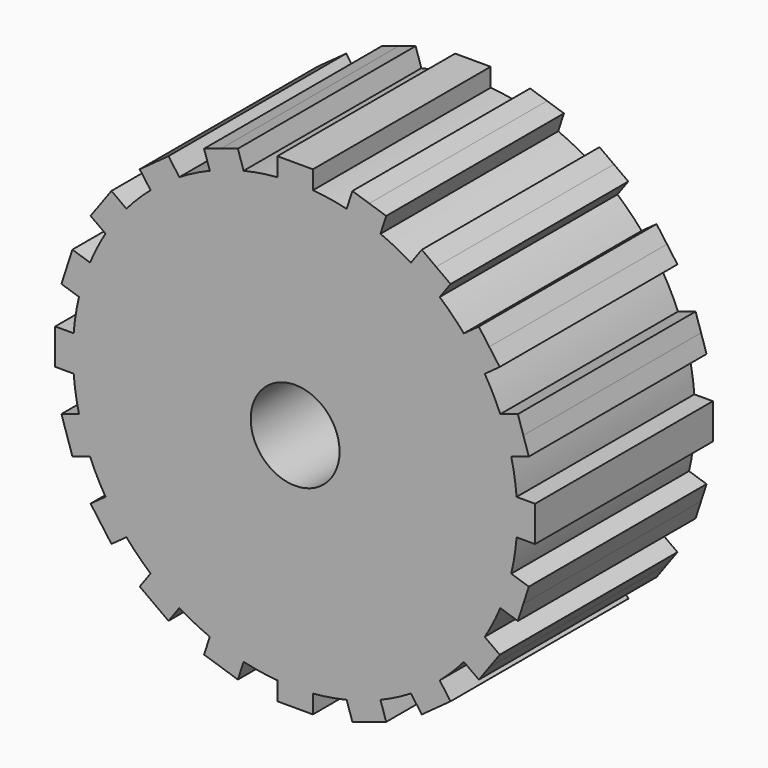
from build123d import *

# Parameters (mm, degrees)
F0_R     = 1.27
F1_DEPTH = 6.35


# Not quite as in the source:
# - a feature names something its author has since deleted; it is built from what else it names


with BuildPart() as f1:
    # F0 (on Front) → F1 (new body)
    with BuildSketch(Plane.XZ):
        with BuildLine():
            ThreePointArc((-2.4391053202, 5.8628717568), (-1.9622579143, 6.0392088785), (-1.4728318996, 6.1768330231))
            Line((-1.4728318996, 6.1768330231), (-1.6361018371, 6.6793262219))
            Line((-1.6361018371, 6.6793262219), (-2.1192385474, 6.5223455888))
            Line((-2.1192385474, 6.5223455888), (-2.6023752577, 6.3653649556))
            Line((-2.6023752577, 6.3653649556), (-2.4391053202, 5.8628717568))
        make_face()
        with BuildLine():
            ThreePointArc((-0.508, 6.3296473835), (-0.2542037711, 6.3449098057), (0, 6.35))
            Line((0, 6.35), (0, 6.858))
            Line((0, 6.858), (-0.508, 6.858))
            Line((-0.508, 6.858), (-0.508, 6.3296473835))
        make_face()
        with BuildLine():
            ThreePointArc((0, 6.35), (0.2542037711, 6.3449098057), (0.508, 6.3296473835))
            Line((0.508, 6.3296473835), (0.508, 6.858))
            Line((0.508, 6.858), (0, 6.858))
            Line((0, 6.858), (0, 6.35))
        make_face()
        with BuildLine():
            ThreePointArc((1.4728318996, 6.1768330231), (1.9622579143, 6.0392088785), (2.4391053202, 5.8628717568))
            Line((2.4391053202, 5.8628717568), (2.6023752577, 6.3653649556))
            Line((2.6023752577, 6.3653649556), (2.1192385474, 6.5223455888))
            Line((2.1192385474, 6.5223455888), (1.6361018371, 6.6793262219))
            Line((1.6361018371, 6.6793262219), (1.4728318996, 6.1768330231))
        make_face()
        with BuildLine():
            ThreePointArc((3.3094927511, 5.4193872099), (3.7324363521, 5.1372579143), (4.1314540174, 4.8221973935))
            Line((4.1314540174, 4.8221973935), (4.4420118934, 5.2496436393))
            Line((4.4420118934, 5.2496436393), (4.0310312602, 5.5482385474))
            Line((4.0310312602, 5.5482385474), (3.6200506271, 5.8468334556))
            Line((3.6200506271, 5.8468334556), (3.3094927511, 5.4193872099))
        make_face()
        with BuildLine():
            ThreePointArc((4.8221973935, 4.1314540174), (5.1372579143, 3.7324363521), (5.4193872099, 3.3094927511))
            Line((5.4193872099, 3.3094927511), (5.8468334556, 3.6200506271))
            Line((5.8468334556, 3.6200506271), (5.5482385474, 4.0310312602))
            Line((5.5482385474, 4.0310312602), (5.2496436393, 4.4420118934))
            Line((5.2496436393, 4.4420118934), (4.8221973935, 4.1314540174))
        make_face()
        with BuildLine():
            Line((0.508, -6.858), (0.508, -6.3296473835))
            ThreePointArc((0.508, -6.3296473835), (0, -6.35), (-0.508, -6.3296473835))
            Line((-0.508, -6.3296473835), (-0.508, -6.858))
            Line((-0.508, -6.858), (0, -6.858))
            Line((0, -6.858), (0.508, -6.858))
        make_face()
        with BuildLine():
            Line((2.6023752577, -6.3653649556), (2.4391053202, -5.8628717568))
            ThreePointArc((2.4391053202, -5.8628717568), (1.9622579143, -6.0392088785), (1.4728318996, -6.1768330231))
            Line((1.4728318996, -6.1768330231), (1.6361018371, -6.6793262219))
            Line((1.6361018371, -6.6793262219), (2.1192385474, -6.5223455888))
            Line((2.1192385474, -6.5223455888), (2.6023752577, -6.3653649556))
        make_face()
        with BuildLine():
            Line((4.4420118934, -5.2496436393), (4.1314540174, -4.8221973935))
            ThreePointArc((4.1314540174, -4.8221973935), (3.7324363521, -5.1372579143), (3.3094927511, -5.4193872099))
            Line((3.3094927511, -5.4193872099), (3.6200506271, -5.8468334556))
            Line((3.6200506271, -5.8468334556), (4.0310312602, -5.5482385474))
            Line((4.0310312602, -5.5482385474), (4.4420118934, -5.2496436393))
        make_face()
        with BuildLine():
            Line((5.8468334556, -3.6200506271), (5.4193872099, -3.3094927511))
            ThreePointArc((5.4193872099, -3.3094927511), (5.1372579143, -3.7324363521), (4.8221973935, -4.1314540174))
            Line((4.8221973935, -4.1314540174), (5.2496436393, -4.4420118934))
            Line((5.2496436393, -4.4420118934), (5.5482385474, -4.0310312602))
            Line((5.5482385474, -4.0310312602), (5.8468334556, -3.6200506271))
        make_face()
        with BuildLine():
            Line((6.6793262219, -1.6361018371), (6.1768330231, -1.4728318996))
            ThreePointArc((6.1768330231, -1.4728318996), (6.0392088785, -1.9622579143), (5.8628717568, -2.4391053202))
            Line((5.8628717568, -2.4391053202), (6.3653649556, -2.6023752577))
            Line((6.3653649556, -2.6023752577), (6.5223455888, -2.1192385474))
            Line((6.5223455888, -2.1192385474), (6.6793262219, -1.6361018371))
        make_face()
        with BuildLine():
            ThreePointArc((6.3296473835, 0.508), (6.3449098057, 0.2542037711), (6.35, 0))
            ThreePointArc((6.35, 0), (6.3449098057, -0.2542037711), (6.3296473835, -0.508))
            Line((6.3296473835, -0.508), (6.858, -0.508))
            Line((6.858, -0.508), (6.858, 0))
            Line((6.858, 0), (6.858, 0.508))
            Line((6.858, 0.508), (6.3296473835, 0.508))
        make_face()
        with BuildLine():
            ThreePointArc((5.8628717568, 2.4391053202), (6.0392088785, 1.9622579143), (6.1768330231, 1.4728318996))
            Line((6.1768330231, 1.4728318996), (6.6793262219, 1.6361018371))
            Line((6.6793262219, 1.6361018371), (6.5223455888, 2.1192385474))
            Line((6.5223455888, 2.1192385474), (6.3653649556, 2.6023752577))
            Line((6.3653649556, 2.6023752577), (5.8628717568, 2.4391053202))
        make_face()
        with BuildLine():
            ThreePointArc((-4.1314540174, 4.8221973935), (-3.7324363521, 5.1372579143), (-3.3094927511, 5.4193872099))
            Line((-3.3094927511, 5.4193872099), (-3.6200506271, 5.8468334556))
            Line((-3.6200506271, 5.8468334556), (-4.0310312602, 5.5482385474))
            Line((-4.0310312602, 5.5482385474), (-4.4420118934, 5.2496436393))
            Line((-4.4420118934, 5.2496436393), (-4.1314540174, 4.8221973935))
        make_face()
        with BuildLine():
            ThreePointArc((-5.4193872099, 3.3094927511), (-5.1372579143, 3.7324363521), (-4.8221973935, 4.1314540174))
            Line((-4.8221973935, 4.1314540174), (-5.2496436393, 4.4420118934))
            Line((-5.2496436393, 4.4420118934), (-5.5482385474, 4.0310312602))
            Line((-5.5482385474, 4.0310312602), (-5.8468334556, 3.6200506271))
            Line((-5.8468334556, 3.6200506271), (-5.4193872099, 3.3094927511))
        make_face()
        with BuildLine():
            ThreePointArc((-6.1768330231, 1.4728318996), (-6.0392088785, 1.9622579143), (-5.8628717568, 2.4391053202))
            Line((-5.8628717568, 2.4391053202), (-6.3653649556, 2.6023752577))
            Line((-6.3653649556, 2.6023752577), (-6.5223455888, 2.1192385474))
            Line((-6.5223455888, 2.1192385474), (-6.6793262219, 1.6361018371))
            Line((-6.6793262219, 1.6361018371), (-6.1768330231, 1.4728318996))
        make_face()
        with BuildLine():
            Line((-6.858, -0.508), (-6.3296473835, -0.508))
            ThreePointArc((-6.3296473835, -0.508), (-6.35, 0), (-6.3296473835, 0.508))
            Line((-6.3296473835, 0.508), (-6.858, 0.508))
            Line((-6.858, 0.508), (-6.858, 0))
            Line((-6.858, 0), (-6.858, -0.508))
        make_face()
        with BuildLine():
            ThreePointArc((6.3296473835, -0.508), (6.3449098057, -0.2542037711), (6.35, 0))
            ThreePointArc((6.35, 0), (6.3449098057, 0.2542037711), (6.3296473835, 0.508))
            ThreePointArc((6.3296473835, 0.508), (6.2718209628, 0.993358853), (6.1768330231, 1.4728318996))
            ThreePointArc((6.1768330231, 1.4728318996), (6.0392088785, 1.9622579143), (5.8628717568, 2.4391053202))
            ThreePointArc((5.8628717568, 2.4391053202), (5.6578914286, 2.8828396733), (5.4193872099, 3.3094927511))
            ThreePointArc((5.4193872099, 3.3094927511), (5.1372579143, 3.7324363521), (4.8221973935, 4.1314540174))
            ThreePointArc((4.8221973935, 4.1314540174), (4.4901280605, 4.4901280605), (4.1314540174, 4.8221973935))
            ThreePointArc((4.1314540174, 4.8221973935), (3.7324363521, 5.1372579143), (3.3094927511, 5.4193872099))
            ThreePointArc((3.3094927511, 5.4193872099), (2.8828396733, 5.6578914286), (2.4391053202, 5.8628717568))
            ThreePointArc((2.4391053202, 5.8628717568), (1.9622579143, 6.0392088785), (1.4728318996, 6.1768330231))
            ThreePointArc((1.4728318996, 6.1768330231), (0.993358853, 6.2718209628), (0.508, 6.3296473835))
            ThreePointArc((0.508, 6.3296473835), (0.2542037711, 6.3449098057), (0, 6.35))
            ThreePointArc((0, 6.35), (-0.2542037711, 6.3449098057), (-0.508, 6.3296473835))
            ThreePointArc((-0.508, 6.3296473835), (-0.993358853, 6.2718209628), (-1.4728318996, 6.1768330231))
            ThreePointArc((-1.4728318996, 6.1768330231), (-1.9622579143, 6.0392088785), (-2.4391053202, 5.8628717568))
            ThreePointArc((-2.4391053202, 5.8628717568), (-2.8828396733, 5.6578914286), (-3.3094927511, 5.4193872099))
            ThreePointArc((-3.3094927511, 5.4193872099), (-3.7324363521, 5.1372579143), (-4.1314540174, 4.8221973935))
            ThreePointArc((-4.1314540174, 4.8221973935), (-4.4901280605, 4.4901280605), (-4.8221973935, 4.1314540174))
            ThreePointArc((-4.8221973935, 4.1314540174), (-5.1372579143, 3.7324363521), (-5.4193872099, 3.3094927511))
            ThreePointArc((-5.4193872099, 3.3094927511), (-5.6578914286, 2.8828396733), (-5.8628717568, 2.4391053202))
            ThreePointArc((-5.8628717568, 2.4391053202), (-6.0392088785, 1.9622579143), (-6.1768330231, 1.4728318996))
            ThreePointArc((-6.1768330231, 1.4728318996), (-6.2718209628, 0.993358853), (-6.3296473835, 0.508))
            ThreePointArc((-6.3296473835, 0.508), (-6.35, 0), (-6.3296473835, -0.508))
            ThreePointArc((-6.3296473835, -0.508), (-6.2718209628, -0.993358853), (-6.1768330231, -1.4728318996))
            ThreePointArc((-6.1768330231, -1.4728318996), (-6.0392088785, -1.9622579143), (-5.8628717568, -2.4391053202))
            ThreePointArc((-5.8628717568, -2.4391053202), (-5.6578914286, -2.8828396733), (-5.4193872099, -3.3094927511))
            ThreePointArc((-5.4193872099, -3.3094927511), (-5.1372579143, -3.7324363521), (-4.8221973935, -4.1314540174))
            ThreePointArc((-4.8221973935, -4.1314540174), (-4.4901280605, -4.4901280605), (-4.1314540174, -4.8221973935))
            ThreePointArc((-4.1314540174, -4.8221973935), (-3.7324363521, -5.1372579143), (-3.3094927511, -5.4193872099))
            ThreePointArc((-3.3094927511, -5.4193872099), (-2.8828396733, -5.6578914286), (-2.4391053202, -5.8628717568))
            ThreePointArc((-2.4391053202, -5.8628717568), (-1.9622579143, -6.0392088785), (-1.4728318996, -6.1768330231))
            ThreePointArc((-1.4728318996, -6.1768330231), (-0.993358853, -6.2718209628), (-0.508, -6.3296473835))
            ThreePointArc((-0.508, -6.3296473835), (0, -6.35), (0.508, -6.3296473835))
            ThreePointArc((0.508, -6.3296473835), (0.993358853, -6.2718209628), (1.4728318996, -6.1768330231))
            ThreePointArc((1.4728318996, -6.1768330231), (1.9622579143, -6.0392088785), (2.4391053202, -5.8628717568))
            ThreePointArc((2.4391053202, -5.8628717568), (2.8828396733, -5.6578914286), (3.3094927511, -5.4193872099))
            ThreePointArc((3.3094927511, -5.4193872099), (3.7324363521, -5.1372579143), (4.1314540174, -4.8221973935))
            ThreePointArc((4.1314540174, -4.8221973935), (4.4901280605, -4.4901280605), (4.8221973935, -4.1314540174))
            ThreePointArc((4.8221973935, -4.1314540174), (5.1372579143, -3.7324363521), (5.4193872099, -3.3094927511))
            ThreePointArc((5.4193872099, -3.3094927511), (5.6578914286, -2.8828396733), (5.8628717568, -2.4391053202))
            ThreePointArc((5.8628717568, -2.4391053202), (6.0392088785, -1.9622579143), (6.1768330231, -1.4728318996))
            ThreePointArc((6.1768330231, -1.4728318996), (6.2718209628, -0.993358853), (6.3296473835, -0.508))
        make_face()
        Circle(F0_R, mode=Mode.SUBTRACT)
        with BuildLine():
            Line((-6.3653649556, -2.6023752577), (-5.8628717568, -2.4391053202))
            ThreePointArc((-5.8628717568, -2.4391053202), (-6.0392088785, -1.9622579143), (-6.1768330231, -1.4728318996))
            Line((-6.1768330231, -1.4728318996), (-6.6793262219, -1.6361018371))
            Line((-6.6793262219, -1.6361018371), (-6.5223455888, -2.1192385474))
            Line((-6.5223455888, -2.1192385474), (-6.3653649556, -2.6023752577))
        make_face()
        with BuildLine():
            Line((-5.2496436393, -4.4420118934), (-4.8221973935, -4.1314540174))
            ThreePointArc((-4.8221973935, -4.1314540174), (-5.1372579143, -3.7324363521), (-5.4193872099, -3.3094927511))
            Line((-5.4193872099, -3.3094927511), (-5.8468334556, -3.6200506271))
            Line((-5.8468334556, -3.6200506271), (-5.5482385474, -4.0310312602))
            Line((-5.5482385474, -4.0310312602), (-5.2496436393, -4.4420118934))
        make_face()
        with BuildLine():
            Line((-3.6200506271, -5.8468334556), (-3.3094927511, -5.4193872099))
            ThreePointArc((-3.3094927511, -5.4193872099), (-3.7324363521, -5.1372579143), (-4.1314540174, -4.8221973935))
            Line((-4.1314540174, -4.8221973935), (-4.4420118934, -5.2496436393))
            Line((-4.4420118934, -5.2496436393), (-4.0310312602, -5.5482385474))
            Line((-4.0310312602, -5.5482385474), (-3.6200506271, -5.8468334556))
        make_face()
        with BuildLine():
            Line((-1.6361018371, -6.6793262219), (-1.4728318996, -6.1768330231))
            ThreePointArc((-1.4728318996, -6.1768330231), (-1.9622579143, -6.0392088785), (-2.4391053202, -5.8628717568))
            Line((-2.4391053202, -5.8628717568), (-2.6023752577, -6.3653649556))
            Line((-2.6023752577, -6.3653649556), (-2.1192385474, -6.5223455888))
            Line((-2.1192385474, -6.5223455888), (-1.6361018371, -6.6793262219))
        make_face()
    extrude(amount=F1_DEPTH)


solid = f1.part
